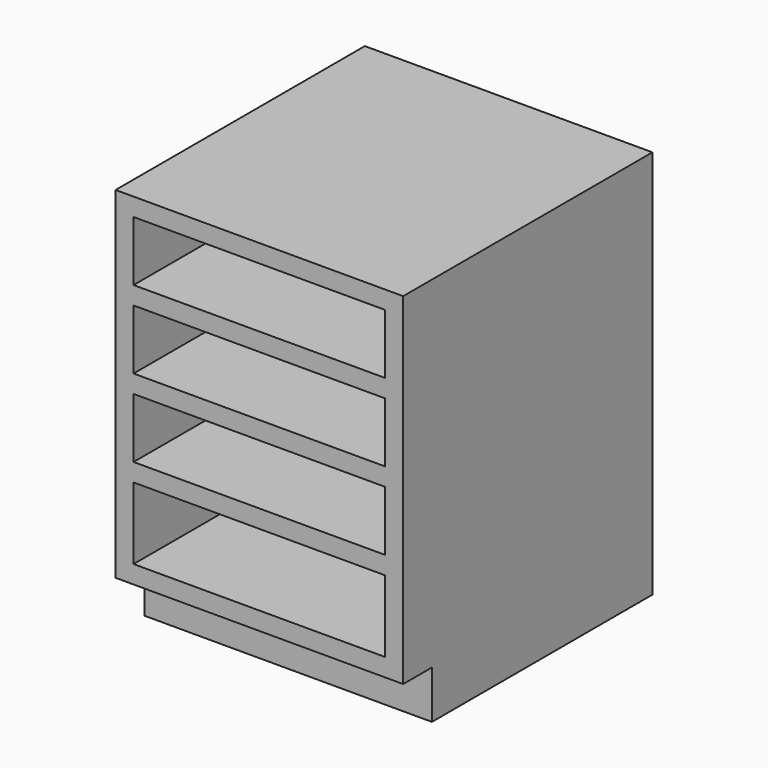
from build123d import *

# Parameters (mm, degrees)
F1_DEPTH = 609.6
F2_W     = 533.4
F2_H     = 127
F2_H_2   = 152.4
F3_DEPTH = 596.9


# Not quite as in the source:
# - a feature names something its author has since deleted; it is built from what else it names


with BuildPart() as f1:
    # F0 (on Right) → F1 (new body)
    with BuildSketch(Plane.YZ):
        Polygon((-584.2, 0), (0, 0), (0, 825.5), (-660.4, 825.5), (-660.4, 101.6), (-584.2, 101.6), align=None)
    extrude(amount=F1_DEPTH)

    # F2 (on face) → F3 (cut)
    with BuildSketch(Plane.XZ.offset(660.4)):
        with Locations((304.8, 723.9)):
            Rectangle(F2_W, F2_H)
        with Locations((304.8, 558.8)):
            Rectangle(F2_W, F2_H)
        with Locations((304.8, 393.7)):
            Rectangle(F2_W, F2_H)
        with Locations((304.8, 215.9)):
            Rectangle(F2_W, F2_H_2)
    extrude(amount=-F3_DEPTH, mode=Mode.SUBTRACT)


solid = f1.part
